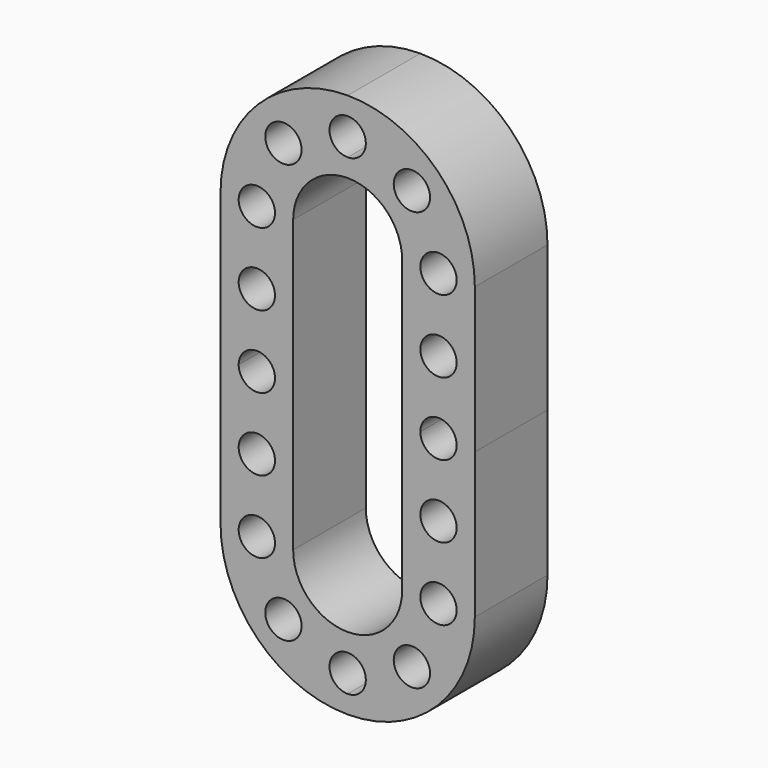
from build123d import *
from build123d import SkipClean  # not in build123d's __all__

# Parameters (mm, degrees)
F0_R     = 5
F1_DEPTH = 25


with BuildPart() as f1:
    # F0 (on Front) → F1 (new body)
    with BuildSketch(Plane.XZ):
        with BuildLine():
            ThreePointArc((-15, 40), (-10.6066017178, 50.6066017178), (0, 55))
            Line((0, 55), (0, 60))
            ThreePointArc((0, 60), (-5, 65), (0, 70))
            Line((0, 70), (0, 75))
            ThreePointArc((0, 75), (-24.7487373415, 64.7487373415), (-35, 40))
            Line((-35, 40), (-35, 0))
            Line((-35, 0), (-30, 0))
            ThreePointArc((-30, 0), (-25, 5), (-20, 0))
            Line((-20, 0), (-15, 0))
            Line((-15, 0), (-15, 40))
        make_face()
        with Locations((-25, 20)):
            Circle(F0_R, mode=Mode.SUBTRACT)
        with Locations((-25, 40)):
            Circle(F0_R, mode=Mode.SUBTRACT)
        with Locations((-17.6776695297, 57.6776695297)):
            Circle(F0_R, mode=Mode.SUBTRACT)
    extrude(amount=F1_DEPTH)

    # F2: F1 across plane


with BuildPart() as f1_1:
    add(f1.part, clean=False)
    with SkipClean():  # cleaning this boolean's faces spoils the solid; the shape is the same uncleaned
        add(f1.part.mirror(Plane.YZ), clean=False)

    # F3: F1 across plane


with BuildPart() as f1_2:
    add(f1_1.part, clean=False)
    add(f1_1.part.mirror(Plane.XY), clean=False)


solid = f1_2.part
